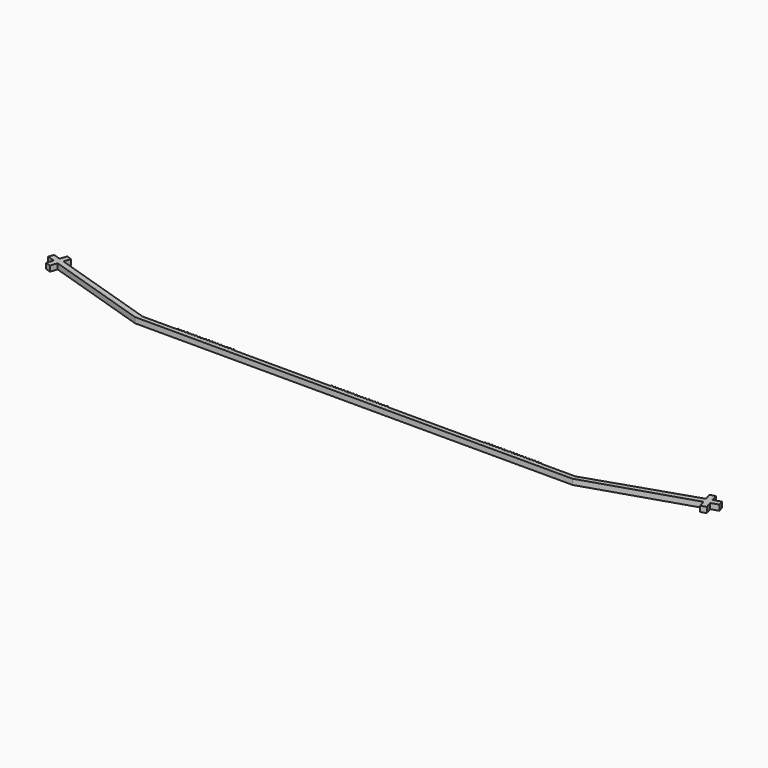
from build123d import *

# Parameters (mm, degrees)
F1_DEPTH = 4.45


# Not quite as in the source:
# - ends of sketch curves that miss each other by under 0.0002 mm in the source are joined


with BuildPart() as f1:
    # F0 (on Top) → F1 (new body)
    with BuildSketch(Plane.XY):
        Polygon((-333.2542810038, 32.8803343494), (-248.602052407, 5.7287194142), (106.997947593, 5.7287194142), (191.6501761898, 32.8803342256), (193.4310519051, 27.3279905247), (197.6684244277, 28.6870983589), (195.8875472553, 34.2394466025), (201.9341350122, 36.1788476693), (200.575027178, 40.4162201919), (194.5284394211, 38.4768191251), (192.747550032, 44.0292054574), (188.5101775095, 42.6700976232), (190.2910668985, 37.1177112909), (106.2874620851, 9.385804846), (78.792851131, 9.385804846), (77.9268646264, 10.5272957241), (77.0608781163, 9.385804846), (76.292851131, 9.385804846), (75.4268646264, 10.5272957241), (74.5608781163, 9.385804846), (73.792851131, 9.385804846), (72.9268646264, 10.5272957241), (72.0608781163, 9.385804846), (71.292851131, 9.385804846), (70.4268646264, 10.5272957241), (69.5608781163, 9.385804846), (68.792851131, 9.385804846), (67.9268646264, 10.5272957241), (67.0608781163, 9.385804846), (66.292851131, 9.385804846), (65.4268646264, 10.5272957241), (64.5608781163, 9.385804846), (63.792851131, 9.385804846), (62.9268646264, 10.5272957241), (62.0608781163, 9.385804846), (61.292851131, 9.385804846), (60.4268646264, 10.5272957241), (59.5608781163, 9.385804846), (58.792851131, 9.385804846), (57.9268646264, 10.5272957241), (57.0608781163, 9.385804846), (56.292851131, 9.385804846), (55.4268646264, 10.5272957241), (54.5608781163, 9.385804846), (53.792851131, 9.385804846), (52.9268646264, 10.5272957241), (52.0608781163, 9.385804846), (51.292851131, 9.385804846), (50.4268646264, 10.5272957241), (49.5608781163, 9.385804846), (48.792851131, 9.385804846), (47.9268646264, 10.5272957241), (47.0608781163, 9.385804846), (46.292851131, 9.385804846), (45.4268646264, 10.5272957241), (44.5608781163, 9.385804846), (43.792851131, 9.385804846), (42.9268646264, 10.5272957241), (42.0608781163, 9.385804846), (41.292851131, 9.385804846), (40.4268646264, 10.5272957241), (39.5608781163, 9.385804846), (38.792851131, 9.385804846), (37.9268646264, 10.5272957241), (37.0608781163, 9.385804846), (36.292851131, 9.385804846), (35.4268646264, 10.5272957241), (34.5608781163, 9.385804846), (33.792851131, 9.385804846), (32.9268646264, 10.5272957241), (32.0608781163, 9.385804846), (-46.207148869, 9.385804846), (-47.0731353736, 10.5272957241), (-47.9391218837, 9.385804846), (-48.707148869, 9.385804846), (-49.5731353736, 10.5272957241), (-50.4391218837, 9.385804846), (-51.207148869, 9.385804846), (-52.0731353736, 10.5272957241), (-52.9391218837, 9.385804846), (-53.707148869, 9.385804846), (-54.5731353736, 10.5272957241), (-55.4391218837, 9.385804846), (-56.207148869, 9.385804846), (-57.0731353736, 10.5272957241), (-57.9391218837, 9.385804846), (-58.707148869, 9.385804846), (-59.5731353736, 10.5272957241), (-60.4391218837, 9.385804846), (-61.207148869, 9.385804846), (-62.0731353736, 10.5272957241), (-62.9391218837, 9.385804846), (-63.707148869, 9.385804846), (-64.5731353736, 10.5272957241), (-65.4391218837, 9.385804846), (-66.207148869, 9.385804846), (-67.0731353736, 10.5272957241), (-67.9391218837, 9.385804846), (-68.707148869, 9.385804846), (-69.5731353736, 10.5272957241), (-70.4391218837, 9.385804846), (-71.207148869, 9.385804846), (-72.0731353736, 10.5272957241), (-72.9391218837, 9.385804846), (-73.707148869, 9.385804846), (-74.5731353736, 10.5272957241), (-75.4391218837, 9.385804846), (-76.207148869, 9.385804846), (-77.0731353736, 10.5272957241), (-77.9391218837, 9.385804846), (-78.707148869, 9.385804846), (-79.5731353736, 10.5272957241), (-80.4391218837, 9.385804846), (-81.207148869, 9.385804846), (-82.0731353736, 10.5272957241), (-82.9391218837, 9.385804846), (-83.707148869, 9.385804846), (-84.5731353736, 10.5272957241), (-85.4391218837, 9.385804846), (-86.207148869, 9.385804846), (-87.0731353736, 10.5272957241), (-87.9391218837, 9.385804846), (-88.707148869, 9.385804846), (-89.5731353736, 10.5272957241), (-90.4391218837, 9.385804846), (-91.207148869, 9.385804846), (-92.0731353736, 10.5272957241), (-92.9391218837, 9.385804846), (-171.207148869, 9.385804846), (-172.0731353736, 10.5272957241), (-172.9391218837, 9.385804846), (-173.707148869, 9.385804846), (-174.5731353736, 10.5272957241), (-175.4391218837, 9.385804846), (-176.207148869, 9.385804846), (-177.0731353736, 10.5272957241), (-177.9391218837, 9.385804846), (-178.707148869, 9.385804846), (-179.5731353736, 10.5272957241), (-180.4391218837, 9.385804846), (-181.207148869, 9.385804846), (-182.0731353736, 10.5272957241), (-182.9391218837, 9.385804846), (-183.707148869, 9.385804846), (-184.5731353736, 10.5272957241), (-185.4391218837, 9.385804846), (-186.207148869, 9.385804846), (-187.0731353736, 10.5272957241), (-187.9391218837, 9.385804846), (-188.707148869, 9.385804846), (-189.5731353736, 10.5272957241), (-190.4391218837, 9.385804846), (-191.207148869, 9.385804846), (-192.0731353736, 10.5272957241), (-192.9391218837, 9.385804846), (-193.707148869, 9.385804846), (-194.5731353736, 10.5272957241), (-195.4391218837, 9.385804846), (-196.207148869, 9.385804846), (-197.0731353736, 10.5272957241), (-197.9391218837, 9.385804846), (-198.707148869, 9.385804846), (-199.5731353736, 10.5272957241), (-200.4391218837, 9.385804846), (-201.207148869, 9.385804846), (-202.0731353736, 10.5272957241), (-202.9391218837, 9.385804846), (-203.707148869, 9.385804846), (-204.5731353736, 10.5272957241), (-205.4391218837, 9.385804846), (-206.207148869, 9.385804846), (-207.0731353736, 10.5272957241), (-207.9391218837, 9.385804846), (-208.707148869, 9.385804846), (-209.5731353736, 10.5272957241), (-210.4391218837, 9.385804846), (-211.207148869, 9.385804846), (-212.0731353736, 10.5272957241), (-212.9391218837, 9.385804846), (-213.707148869, 9.385804846), (-214.5731353736, 10.5272957241), (-215.4391218837, 9.385804846), (-216.207148869, 9.385804846), (-217.0731353736, 10.5272957241), (-217.9391218837, 9.385804846), (-245.4337328672, 9.385804846), (-247.2429431158, 9.9660964794), (-331.8951717126, 37.1177114147), (-330.1142823235, 42.6700977471), (-334.3516548461, 44.0292055813), (-336.1325442352, 38.4768192489), (-342.1791319921, 40.4162203157), (-343.5382398263, 36.1788477931), (-337.4916520694, 34.2394467263), (-339.2725292417, 28.6870984827), (-335.0351567192, 27.3279906485), align=None)
    extrude(amount=F1_DEPTH)


solid = f1.part
